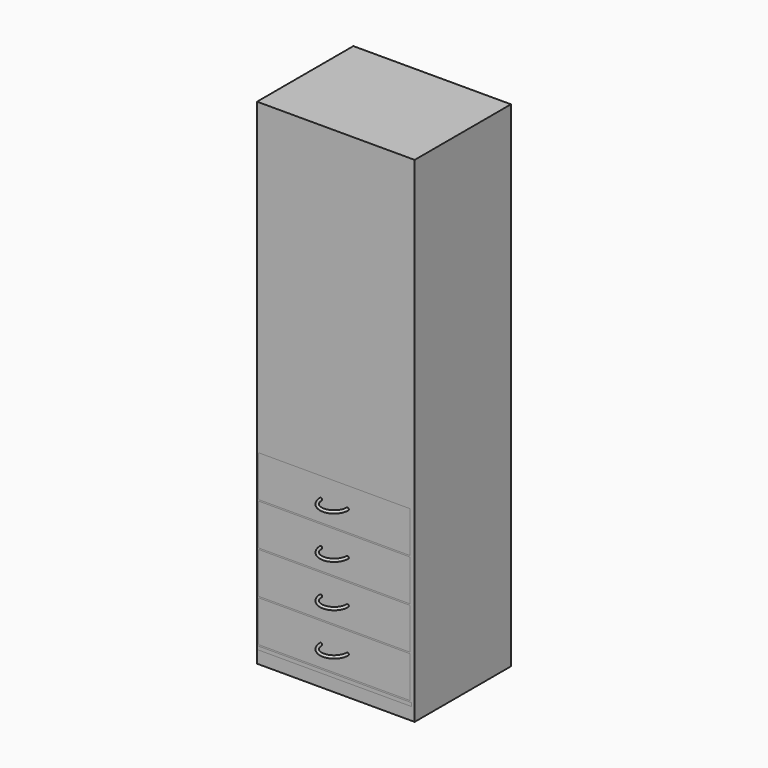
from build123d import *

# Parameters (mm, degrees)
F0_W      = 736.6
F0_H      = 15.875
F1_DEPTH  = 2362.2
F2_DEPTH  = 2362.2
F0_W_2    = 15.875
F0_H_2    = 542.925
F3_DEPTH  = 2362.2
F4_DEPTH  = 59.055
F5_START  = 59.69
F5_DEPTH  = 16.51
F7_START  = 6.35
F6_W      = 15.875
F6_H      = 527.05
F6_H_2    = 15.875
F6_W_2    = 692.150006336
F7_DEPTH  = 196.85
F8_START  = 6.35
F8_DEPTH  = 15.875
F12_DEPTH = 25.4
F13_START = 895.35
F13_DEPTH = 15.875
F14_START = 909.955
F14_DEPTH = 17.145
F15_START = 2346.325
F15_DEPTH = 15.875
F16_R     = 6.35
F17_ANGLE = 180
F22_START = -15.875
F21_R     = 9.525
F22_DEPTH = 720.725


# Not quite as in the source:
# - a feature names something its author has since deleted; it is built from what else it names


with BuildPart() as f1:
    # F0 (on Top) → F1 (new body)
    with BuildSketch(Plane.XY):
        with Locations((120.5184794962, -234.8712890148)):
            Rectangle(F0_W, F0_H)
    extrude(amount=F1_DEPTH)



with BuildPart() as f2:
    # F0 (on Top) → F2 (new body)
    with BuildSketch(Plane.XY):
        Polygon((504.6934794962, 331.8662109852), (-247.7815205038, 331.8662109852), (-247.7815205038, 315.9912109852), (488.8184794962, 315.9912109852), (504.6934794962, 315.9912109852), align=None)
    extrude(amount=F2_DEPTH)


with BuildPart() as f1_1:
    add(f1.part)

    add(f2.part)  # F3 merges F2
    # F0 (on Top) → F3 (join)
    with BuildSketch(Plane.XY):
        Polygon((504.6934794962, 331.8662109852), (-247.7815205038, 331.8662109852), (-247.7815205038, 315.9912109852), (488.8184794962, 315.9912109852), (504.6934794962, 315.9912109852), align=None)
        with Locations((496.7559794962, 44.5287109852)):
            Rectangle(F0_W_2, F0_H_2)
        with Locations((496.7559794962, -234.8712890148)):
            Rectangle(F0_W_2, F0_H)
    extrude(amount=F3_DEPTH)

    # F0 (on Top) → F4 (join)
    with BuildSketch(Plane.XY):
        with Locations((120.5184794962, -234.8712890148)):
            Rectangle(F0_W, F0_H)
    extrude(amount=F4_DEPTH)

    # F0 (on Top) → F12 (join)
    with BuildSketch(Plane.XY):
        with Locations((120.5184794962, 44.5287109852)):
            Rectangle(F0_W, F0_H_2)
        with Locations((120.5184794962, -234.8712890148)):
            Rectangle(F0_W, F0_H)
    extrude(amount=F12_DEPTH)

    # F0 (on Top) → F13 (join)
    with BuildSketch(Plane.XY.offset(F13_START)):
        with Locations((120.5184794962, 44.5287109852)):
            Rectangle(F0_W, F0_H_2)
        with Locations((120.5184794962, -234.8712890148)):
            Rectangle(F0_W, F0_H)
    extrude(amount=F13_DEPTH)

    # F0 (on Top) → F14 (join)
    with BuildSketch(Plane.XY.offset(F14_START)):
        with Locations((120.5184794962, 44.5287109852)):
            Rectangle(F0_W, F0_H_2)
        with Locations((120.5184794962, -234.8712890148)):
            Rectangle(F0_W, F0_H)
    extrude(amount=F14_DEPTH)

    # F0 (on Top) → F15 (join)
    with BuildSketch(Plane.XY.offset(F15_START)):
        with Locations((120.5184794962, -234.8712890148)):
            Rectangle(F0_W, F0_H)
        with Locations((120.5184794962, 44.5287109852)):
            Rectangle(F0_W, F0_H_2)
    extrude(amount=F15_DEPTH)


with BuildPart() as f5:
    # F0 (on Top) → F5 (new body)
    with BuildSketch(Plane.XY.offset(F5_START)):
        with Locations((120.5184794962, 44.5287109852)):
            Rectangle(F0_W, F0_H_2)
        with Locations((120.5184794962, -234.8712890148)):
            Rectangle(F0_W, F0_H)
    extrude(amount=F5_DEPTH)


with BuildPart() as f7:
    # F6 (on face) → F7 (new body)
    with BuildSketch(Plane.XY.offset(76.2).offset(F7_START)):
        with Locations((-233.4940205038, 36.5912109852)):
            Rectangle(F6_W, F6_H)
        with Locations((-233.4940205038, 308.0537109852)):
            Rectangle(F6_W, F6_H_2)
        with Locations((120.5184826642, 308.0537109852)):
            Rectangle(F6_W_2, F6_H_2)
        with Locations((-233.4940205038, -234.8712890148)):
            Rectangle(F6_W, F6_H_2)
        with Locations((120.5184826642, -234.8712890148)):
            Rectangle(F6_W_2, F6_H_2)
        with Locations((474.5309858322, 308.0537109852)):
            Rectangle(F6_W, F6_H_2)
        with Locations((474.5309858322, 36.5912109852)):
            Rectangle(F6_W, F6_H)
        with Locations((474.5309858322, -234.8712890148)):
            Rectangle(F6_W, F6_H_2)
    extrude(amount=F7_DEPTH)

    # F6 (on face) → F8 (join)
    with BuildSketch(Plane.XY.offset(76.2).offset(F8_START)):
        with Locations((120.5184826642, 36.5912109852)):
            Rectangle(F6_W_2, F6_H)
    extrude(amount=F8_DEPTH)


with BuildPart() as f9_1:
    # F9: copy of F7
    add(f7.part.moved(Location((0, 0, 203.2))))


with BuildPart() as f10_1:
    # F10: copy of F9_1
    add(f9_1.part.moved(Location((0, 0, 203.2))))


with BuildPart() as f11_1:
    # F11: copy of F10_1
    add(f10_1.part.moved(Location((0, 0, 203.2))))


with BuildPart() as f17:
    # F16 (on face) → F17 (revolve)
    with BuildSketch(Plane.XZ.offset(242.8087890148)):
        with Locations((57.0184826642, 180.975)):
            Circle(F16_R)
    revolve(axis=Axis((120.5184826642, -242.8087890148, 180.975), (0, 0, 1)), revolution_arc=F17_ANGLE)


with BuildPart() as f18_1:
    # F18: copy of F17
    add(f17.part.moved(Location((0, 0, 203.2))))


with BuildPart() as f19_1:
    # F19: copy of F18_1
    add(f18_1.part.moved(Location((0, 0, 203.2))))


with BuildPart() as f20_1:
    # F20: copy of F19_1
    add(f19_1.part.moved(Location((0, 0, 203.2))))


with BuildPart() as f22:
    # F21 (on face) → F22 (new body)
    with BuildSketch(Plane.YZ.offset(504.6934794962).offset(F22_START)):
        with Locations((30.24783488, 2260.6)):
            Circle(F21_R)
    extrude(amount=-F22_DEPTH)


solid = Compound([f1_1.part, f5.part, f7.part, f9_1.part, f10_1.part, f11_1.part, f17.part, f18_1.part, f19_1.part, f20_1.part, f22.part])
